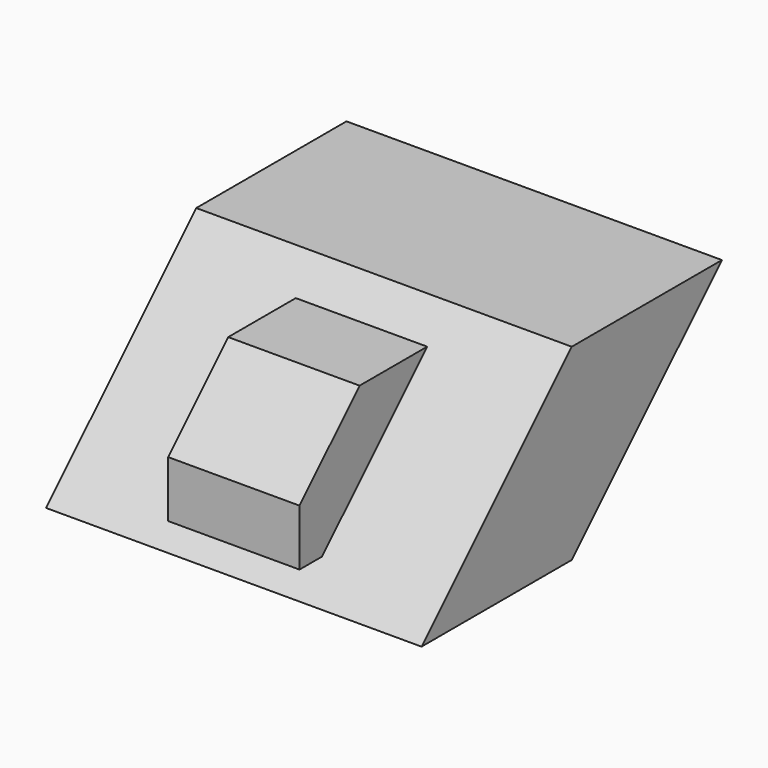
from build123d import *

# Parameters (mm, degrees)
F0_W     = 25.4
F0_H     = 12.7
F1_DEPTH = 25.4
F2_SIZE  = 12.69999
F3_W     = 8.89
F3_H     = 8.89
F4_DEPTH = 25.4
F5_W     = 5.08
F5_H     = 5.08
F6_DEPTH = 3.81
F7_SIZE  = 5.08


# Not quite as in the source:
# - a fillet or chamfer is up to 0.001 mm smaller than in the source, because OpenCascade refuses the exact size


with BuildPart() as f1:
    # F0 (on Front) → F1 (new body)
    with BuildSketch(Plane.XZ):
        with Locations((-12.7, 6.35)):
            Rectangle(F0_W, F0_H)
    extrude(amount=F1_DEPTH)

    # F2 (size 12.7 in the source; OpenCascade refuses exactly that, so slightly less here)
    f2_edges = [f1.edges().sort_by_distance(p)[0] for p in [
        (-12.7, -25.4, 12.7),
        (-12.7, 0, 0),
    ]]
    chamfer(f2_edges, length=F2_SIZE)


with BuildPart() as f4:
    # F3 (on Front) → F4 (new body)
    with BuildSketch(Plane.XZ):
        with Locations((-12.7, 6.35)):
            Rectangle(F3_W, F3_H)
    extrude(amount=F4_DEPTH)

    # F5 (on face) → F6 (cut)
    with BuildSketch(Plane.XZ):
        with Locations((-12.6871485263, 6.3475929201)):
            Rectangle(F5_W, F5_H)
    extrude(amount=F6_DEPTH, mode=Mode.SUBTRACT)

    # F7
    f7_edges = [f4.edges().sort_by_distance(p)[0] for p in [
        (-12.7, -25.4, 10.795),
    ]]
    chamfer(f7_edges, length=F7_SIZE)


solid = Compound([f1.part, f4.part])
